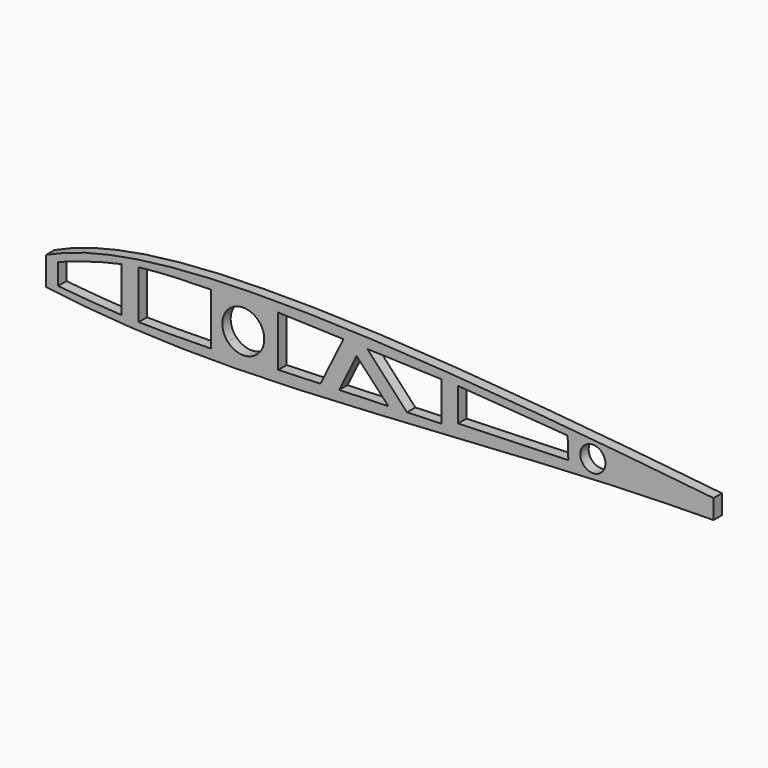
from build123d import *

# Parameters (mm, degrees)
F2_DEPTH = 2.5
F1_R     = 3
F3_DEPTH = 2.5
F5_DEPTH = 2.5
F6_DEPTH = 2.5
F7_DEPTH = 2.5
F8_DEPTH = 2.5
F9_DEPTH = 2.5


# Not quite as in the source:
# - a feature names something its author has since deleted; it is built from what else it names


with BuildPart() as f2:
    # F0 (on Front) → F2 (new body)
    with BuildSketch(Plane.XZ):
        with BuildLine():
            add(Edge.make_bspline(
                [(-96.9805282175, -0.8100506688), (-84.7869920978, 5.1468541776), (-38.6381415733, 10.9636146396), (42.6881882799, 2.4723259958), (100, -4.047003109)],
                knots=[0, 0, 0, 0, 0.374886421, 1, 1, 1, 1], degree=3))
            add(Edge.make_bspline(
                [(-97.5447368223, -7.1186651935), (-99.939251346, -6.5508492693), (-102.885147974, -5.168950634), (-100.0067471137, -2.3789404522), (-96.9805282175, -0.8100506688)],
                knots=[0.0564585679, 0.0564585679, 0.0564585679, 0.0564585679, 0.4847104148, 1, 1, 1, 1], degree=3))
            add(Edge.make_bspline(
                [(-96.5428845142, -7.3406707446), (-96.8949965543, -7.2673488468), (-97.22905608, -7.1935231869), (-97.5447368223, -7.1186651935)],
                knots=[0, 0, 0, 0, 0.0564585679, 0.0564585679, 0.0564585679, 0.0564585679], degree=3))
            add(Edge.make_bspline(
                [(-96.5428845142, -7.3406707446), (-80.7020161693, -9.4302402111), (-44.2471235075, -11.1181020976), (41.8622965332, -3.5518856086), (82.0915186506, -4.6802794425), (100, -4.047003109)],
                knots=[0, 0, 0, 0, 0.2987594418, 0.6837410955, 1, 1, 1, 1], degree=3))
        make_face()
        with BuildLine():
            add(Edge.make_bspline(
                [(-99.8196757147, -4.047003109), (-99.3821638101, -3.2227137691), (-97.9006497107, -2.3042858417), (-96.3385477662, -1.6362179573)],
                knots=[0.5425000514, 0.5425000514, 0.5425000514, 0.5425000514, 1, 1, 1, 1], degree=3))
            add(Edge.make_bspline(
                [(-96.3385477662, -1.6362179573), (-85.7442874691, 3.2900694446), (-38.7960585931, 10.0747672146), (36.943279708, 1.696590452), (86.094097513, -3.3751911245)],
                knots=[0, 0, 0, 0, 0.384923117, 1, 1, 1, 1], degree=3))
            add(Edge.make_bspline(
                [(-97.3825784566, -6.0471531808), (-82.3468325761, -8.841713568), (-44.2551066449, -8.6286827794), (40.9195716837, -3.3120714751), (72.7341022162, -3.1550192186), (86.094097513, -3.3751911245)],
                knots=[0, 0, 0, 0, 0.3131273629, 0.7122131732, 1, 1, 1, 1], degree=3))
            add(Edge.make_bspline(
                [(-97.3825784566, -6.0471531808), (-98.6588937786, -5.8946130057), (-100.1661659123, -5.1778479876), (-99.9138553768, -4.2244412327), (-99.8196757147, -4.047003109)],
                knots=[0, 0, 0, 0, 0.4440177242, 0.5425000514, 0.5425000514, 0.5425000514, 0.5425000514], degree=3))
        make_face(mode=Mode.SUBTRACT)
        with BuildLine():
            add(Edge.make_bspline(
                [(-96.3385477662, -1.6362179573), (-85.7442874691, 3.2900694446), (-38.7960585931, 10.0747672146), (36.943279708, 1.696590452), (86.094097513, -3.3751911245)],
                knots=[0, 0, 0, 0, 0.384923117, 1, 1, 1, 1], degree=3))
            add(Edge.make_bspline(
                [(-99.8196757147, -4.047003109), (-99.3821638101, -3.2227137691), (-97.9006497107, -2.3042858417), (-96.3385477662, -1.6362179573)],
                knots=[0.5425000514, 0.5425000514, 0.5425000514, 0.5425000514, 1, 1, 1, 1], degree=3))
            add(Edge.make_bspline(
                [(-97.3825784566, -6.0471531808), (-98.6588937786, -5.8946130057), (-100.1661659123, -5.1778479876), (-99.9138553768, -4.2244412327), (-99.8196757147, -4.047003109)],
                knots=[0, 0, 0, 0, 0.4440177242, 0.5425000514, 0.5425000514, 0.5425000514, 0.5425000514], degree=3))
            add(Edge.make_bspline(
                [(-97.3825784566, -6.0471531808), (-82.3468325761, -8.841713568), (-44.2551066449, -8.6286827794), (40.9195716837, -3.3120714751), (72.7341022162, -3.1550192186), (86.094097513, -3.3751911245)],
                knots=[0, 0, 0, 0, 0.3131273629, 0.7122131732, 1, 1, 1, 1], degree=3))
        make_face()
        with BuildLine():
            add(Edge.make_bspline(
                [(-96.5428845142, -7.3406707446), (-96.8949965543, -7.2673488468), (-97.22905608, -7.1935231869), (-97.5447368223, -7.1186651935)],
                knots=[0, 0, 0, 0, 0.0564585679, 0.0564585679, 0.0564585679, 0.0564585679], degree=3))
            ThreePointArc((-97.5447368223, -7.1186651935), (-97.052492706, -7.2688477084), (-96.5428845142, -7.3406707446))
        make_face()
    extrude(amount=F2_DEPTH)


with BuildPart() as f2b:
    # F1 (on Front) → F2, piece 2 (new body)
    with BuildSketch(Plane.XZ):
        with Locations((33.7789729238, -1.0305350879)):
            Circle(F1_R)
    extrude(amount=F2_DEPTH)


with BuildPart() as f2c:
    # F1 (on Front) → F2, piece 3 (new body)
    with BuildSketch(Plane.XZ):
        with BuildLine():
            ThreePointArc((-44.542362095, -1.3708024857), (-51.3662704709, 3.2846629299), (-53.2117053896, -4.7672594318))
            Line((-53.2117053896, -4.7672594318), (-45.8404576082, -4.7317403266))
            ThreePointArc((-45.8404576082, -4.7317403266), (-44.8781621403, -3.1722571154), (-44.542362095, -1.3708024857))
        make_face()
        with BuildLine():
            Line((-45.8404576082, -4.7317403266), (-53.2117053896, -4.7672594318))
            ThreePointArc((-53.2117053896, -4.7672594318), (-49.5182693675, -6.3707444394), (-45.8404576082, -4.7317403266))
        make_face()
    extrude(amount=F2_DEPTH)


with BuildPart() as f3_tool:
    # F1 (on Front) → F3 (new body)
    with BuildSketch(Plane.XZ):
        with BuildLine():
            ThreePointArc((-44.542362095, -1.3708024857), (-51.3662704709, 3.2846629299), (-53.2117053896, -4.7672594318))
            Line((-53.2117053896, -4.7672594318), (-45.8404576082, -4.7317403266))
            ThreePointArc((-45.8404576082, -4.7317403266), (-44.8781621403, -3.1722571154), (-44.542362095, -1.3708024857))
        make_face()
        with BuildLine():
            Line((-45.8404576082, -4.7317403266), (-53.2117053896, -4.7672594318))
            ThreePointArc((-53.2117053896, -4.7672594318), (-49.5182693675, -6.3707444394), (-45.8404576082, -4.7317403266))
        make_face()
        with Locations((33.7789729238, -1.0305350879)):
            Circle(F1_R)
    extrude(amount=F3_DEPTH)


with BuildPart() as f2_1:
    add(f2.part)

    # F3: cut by f3_tool
    add(f3_tool.part, mode=Mode.SUBTRACT)

    # F4 (on face) → F5 (cut)
    with BuildSketch(Plane.XZ.offset(2.5)):
        with BuildLine():
            Line((-96.5428845142, -7.3406707446), (-96.5428845142, -0.5989118026))
            add(Edge.make_bspline(
                [(-96.9805282175, -0.8100506688), (-96.8353706427, -0.7391368787), (-96.6894893165, -0.6687582494), (-96.5428845142, -0.5989118026)],
                knots=[0, 0, 0, 0, 0.0044628238, 0.0044628238, 0.0044628238, 0.0044628238], degree=3))
            add(Edge.make_bspline(
                [(-96.9805282175, -0.8100506688), (-100.0067471137, -2.3789404522), (-102.885147974, -5.168950634), (-99.939251346, -6.5508492693), (-97.5447368223, -7.1186651935)],
                knots=[0.0564585679, 0.0564585679, 0.0564585679, 0.0564585679, 0.5717481532, 1, 1, 1, 1], degree=3))
            ThreePointArc((-97.5447368223, -7.1186651935), (-97.052492706, -7.2688477084), (-96.5428845142, -7.3406707446))
        make_face()
    extrude(amount=-F5_DEPTH, mode=Mode.SUBTRACT)

    # F4 (on face) → F6 (cut)
    with BuildSketch(Plane.XZ.offset(2.5)):
        with BuildLine():
            Line((-78.6215588156, -7.3670944992), (-78.6215588156, 3.2958948603))
            add(Edge.make_bspline(
                [(-78.6215588156, 3.2958948603), (-83.9345486349, 2.2532028855), (-88.8194569144, 0.5548157735), (-93.7043651938, -1.1435713386)],
                knots=[0.554896308, 0.554896308, 0.554896308, 0.554896308, 1, 1, 1, 1], degree=3))
            Line((-93.7043651938, -1.1435713386), (-93.7043651938, -6.1954581179))
            add(Edge.make_bspline(
                [(-78.6215588156, -7.3670944992), (-83.7013643272, -7.1077100258), (-88.7028647605, -6.6515840718), (-93.7043651938, -6.1954581179)],
                knots=[0.5793594661, 0.5793594661, 0.5793594661, 0.5793594661, 1, 1, 1, 1], degree=3))
        make_face()
        with BuildLine():
            Line((-57.251535356, -7.4831936508), (-57.251535356, 4.8988820054))
            add(Edge.make_bspline(
                [(-57.251535356, 4.8988820054), (-63.1249518816, 4.7812850577), (-68.9983684072, 4.66368811), (-74.4892291338, 3.9601280834)],
                knots=[0, 0, 0, 0, 0.4418705618, 0.4418705618, 0.4418705618, 0.4418705618], degree=3))
            Line((-74.4892291338, 3.9601280834), (-74.4892291338, -7.5306241193))
            add(Edge.make_bspline(
                [(-57.251535356, -7.4831936508), (-63.0319736557, -7.5857864832), (-68.8124119553, -7.6883793156), (-74.4892291338, -7.5306241193)],
                knots=[0, 0, 0, 0, 0.4658094847, 0.4658094847, 0.4658094847, 0.4658094847], degree=3))
        make_face()
        Polygon((27.7735989974, 1.9125135442), (1.6607665457, 3.840460399), (1.6607665457, -4.047003109), (27.9367215699, -3.2103169474), align=None)
    extrude(amount=-F6_DEPTH, mode=Mode.SUBTRACT)

    # F4 (on face) → F7 (cut)
    with BuildSketch(Plane.XZ.offset(2.5)):
        with BuildLine():
            add(Edge.make_bspline(
                [(62.5460875734, 0.1020588345), (74.6514883615, -1.1873862537), (87.1633646635, -2.586811085), (100, -4.047003109)],
                knots=[0.8599877614, 0.8599877614, 0.8599877614, 0.8599877614, 1, 1, 1, 1], degree=3))
            Line((62.5460875734, 0.1020588345), (62.5460875734, -4.518638291))
            add(Edge.make_bspline(
                [(62.5460875734, -4.518638291), (75.9097127299, -4.3829595873), (88.0075171585, -4.4710790211), (100, -4.047003109)],
                knots=[0.7882160183, 0.7882160183, 0.7882160183, 0.7882160183, 1, 1, 1, 1], degree=3))
        make_face()
    extrude(amount=-F7_DEPTH, mode=Mode.SUBTRACT)

    # F4 (on face) → F8 (cut)
    with BuildSketch(Plane.XZ.offset(2.5)):
        with BuildLine():
            Line((-78.6215588156, -7.3670944992), (-78.6215588156, 3.2958948603))
            add(Edge.make_bspline(
                [(-78.6215588156, 3.2958948603), (-83.9345486349, 2.2532028855), (-88.8194569144, 0.5548157735), (-93.7043651938, -1.1435713386)],
                knots=[0.554896308, 0.554896308, 0.554896308, 0.554896308, 1, 1, 1, 1], degree=3))
            Line((-93.7043651938, -1.1435713386), (-93.7043651938, -6.1954581179))
            add(Edge.make_bspline(
                [(-78.6215588156, -7.3670944992), (-83.7013643272, -7.1077100258), (-88.7028647605, -6.6515840718), (-93.7043651938, -6.1954581179)],
                knots=[0.5793594661, 0.5793594661, 0.5793594661, 0.5793594661, 1, 1, 1, 1], degree=3))
        make_face()
        with BuildLine():
            Line((-57.251535356, -7.4831936508), (-57.251535356, 4.8988820054))
            add(Edge.make_bspline(
                [(-57.251535356, 4.8988820054), (-63.1249518816, 4.7812850577), (-68.9983684072, 4.66368811), (-74.4892291338, 3.9601280834)],
                knots=[0, 0, 0, 0, 0.4418705618, 0.4418705618, 0.4418705618, 0.4418705618], degree=3))
            Line((-74.4892291338, 3.9601280834), (-74.4892291338, -7.5306241193))
            add(Edge.make_bspline(
                [(-57.251535356, -7.4831936508), (-63.0319736557, -7.5857864832), (-68.8124119553, -7.6883793156), (-74.4892291338, -7.5306241193)],
                knots=[0, 0, 0, 0, 0.4658094847, 0.4658094847, 0.4658094847, 0.4658094847], degree=3))
        make_face()
        Polygon((-41.2043631077, 5.3020771593), (-41.2043631077, -6.7306268347), (-31.1431517353, -6.3803097993), (-25.6712666077, 4.7633535934), align=None)
        Polygon((27.7735989974, 1.9125135442), (1.6607665457, 3.840460399), (1.6607665457, -4.047003109), (27.9367215699, -3.2103169474), align=None)
    extrude(amount=-F8_DEPTH, mode=Mode.SUBTRACT)

    # F4 (on face) → F9 (cut)
    with BuildSketch(Plane.XZ.offset(2.5)):
        Polygon((-22.5247312337, 2.2527640685), (-26.6876633679, -6.2251760467), (-14.952923861, -5.8165891476), align=None)
        Polygon((-2.2568607237, 3.9512880641), (-19.9629371484, 4.5653755791), (-10.5242531862, -5.6623891488), (-2.2568607237, -5.3745303303), align=None)
        Polygon((27.7735989974, 1.9125135442), (1.6607665457, 3.840460399), (1.6607665457, -4.047003109), (27.9367215699, -3.2103169474), align=None)
        with BuildLine():
            Line((-57.251535356, -7.4831936508), (-57.251535356, 4.8988820054))
            add(Edge.make_bspline(
                [(-57.251535356, 4.8988820054), (-63.1249518816, 4.7812850577), (-68.9983684072, 4.66368811), (-74.4892291338, 3.9601280834)],
                knots=[0, 0, 0, 0, 0.4418705618, 0.4418705618, 0.4418705618, 0.4418705618], degree=3))
            Line((-74.4892291338, 3.9601280834), (-74.4892291338, -7.5306241193))
            add(Edge.make_bspline(
                [(-57.251535356, -7.4831936508), (-63.0319736557, -7.5857864832), (-68.8124119553, -7.6883793156), (-74.4892291338, -7.5306241193)],
                knots=[0, 0, 0, 0, 0.4658094847, 0.4658094847, 0.4658094847, 0.4658094847], degree=3))
        make_face()
        with BuildLine():
            Line((-78.6215588156, -7.3670944992), (-78.6215588156, 3.2958948603))
            add(Edge.make_bspline(
                [(-78.6215588156, 3.2958948603), (-83.9345486349, 2.2532028855), (-88.8194569144, 0.5548157735), (-93.7043651938, -1.1435713386)],
                knots=[0.554896308, 0.554896308, 0.554896308, 0.554896308, 1, 1, 1, 1], degree=3))
            Line((-93.7043651938, -1.1435713386), (-93.7043651938, -6.1954581179))
            add(Edge.make_bspline(
                [(-78.6215588156, -7.3670944992), (-83.7013643272, -7.1077100258), (-88.7028647605, -6.6515840718), (-93.7043651938, -6.1954581179)],
                knots=[0.5793594661, 0.5793594661, 0.5793594661, 0.5793594661, 1, 1, 1, 1], degree=3))
        make_face()
        Polygon((-41.2043631077, 5.3020771593), (-41.2043631077, -6.7306268347), (-31.1431517353, -6.3803097993), (-25.6712666077, 4.7633535934), align=None)
    extrude(amount=-F9_DEPTH, mode=Mode.SUBTRACT)


with BuildPart() as f2b_1:
    add(f2b.part)

    # F3: cut by f3_tool
    add(f3_tool.part, mode=Mode.SUBTRACT)


with BuildPart() as f2c_1:
    add(f2c.part)

    # F3: cut by f3_tool
    add(f3_tool.part, mode=Mode.SUBTRACT)


solid = f2_1.part
